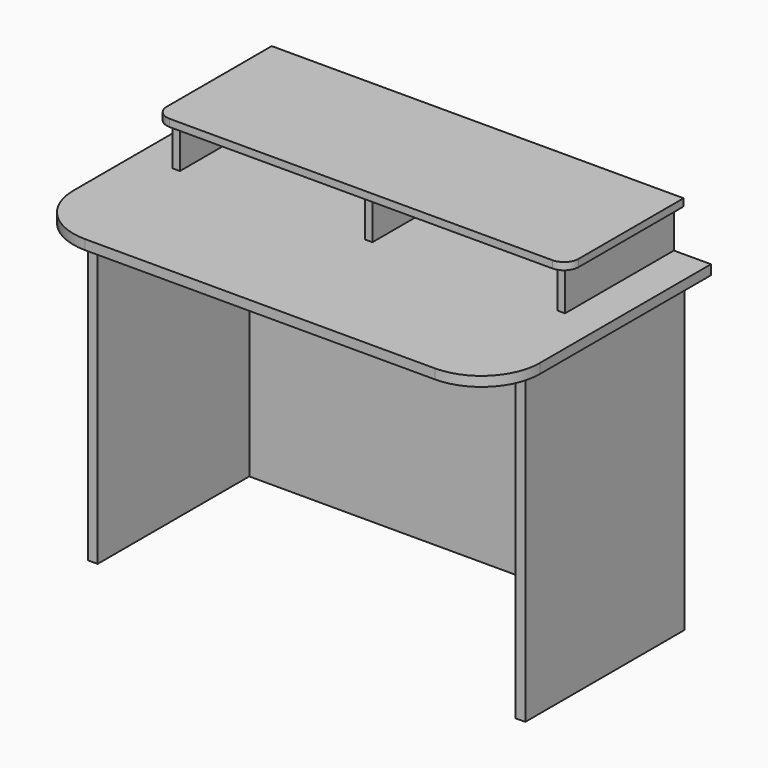
from build123d import *

# Parameters (mm, degrees)
F0_W      = 1219.2
F0_H      = 711.2
F1_DEPTH  = 25.4
F3_DEPTH  = 25.4
F4_W      = 19.05
F4_H      = 355.6
F5_DEPTH  = 109.5375
F6_W      = 1092.2
F6_H      = 25.4
F7_DEPTH  = 812.8
F8_W      = 19.05
F8_H      = 355.6
F9_DEPTH  = 19.05
F10_R     = 38.1
F11_W     = 203.2
F11_H     = 254
F12_DEPTH = 25.4
F13_R     = 25.4


# Not quite as in the source:
# - a feature names something its author has since deleted; it is built from what else it names


with BuildPart() as f1:
    # F0 (on Top) → F1 (new body)
    with BuildSketch(Plane.XY):
        with Locations((609.6, 355.6)):
            Rectangle(F0_W, F0_H)
    extrude(amount=F1_DEPTH)

    # F2 (on face) → F3 (cut)
    with BuildSketch(Plane.XY.offset(25.4)):
        with BuildLine():
            ThreePointArc((152.4, 0), (44.6369265472, 44.6369265472), (0, 152.4))
            Line((0, 152.4), (0, 0))
            Line((0, 0), (152.4, 0))
        make_face()
        with BuildLine():
            ThreePointArc((1219.2, 152.4), (1174.5630734528, 44.6369265472), (1066.8, 0))
            Line((1066.8, 0), (1219.2, 0))
            Line((1219.2, 0), (1219.2, 152.4))
        make_face()
    extrude(amount=-F3_DEPTH, mode=Mode.SUBTRACT)


with BuildPart() as f5:
    # F4 (on face) → F5 (new body)
    with BuildSketch(Plane.XY.offset(25.4)):
        with Locations((106.3625, 533.4)):
            Rectangle(F4_W, F4_H)
    extrude(amount=F5_DEPTH)


with BuildPart() as f5b:
    # F4 (on face) → F5, piece 2 (new body)
    with BuildSketch(Plane.XY.offset(25.4)):
        with Locations((609.6, 533.4)):
            Rectangle(F4_W, F4_H)
    extrude(amount=F5_DEPTH)


with BuildPart() as f5c:
    # F4 (on face) → F5, piece 3 (new body)
    with BuildSketch(Plane.XY.offset(25.4)):
        with Locations((1112.8375, 533.4)):
            Rectangle(F4_W, F4_H)
    extrude(amount=F5_DEPTH)


with BuildPart() as f7:
    # F6 (on face) → F7 (new body)
    with BuildSketch(Plane(origin=(0, 0, 0), x_dir=(1, 0, 0), z_dir=(0, 0, -1))):
        Polygon((63.5, -152.4), (38.1, -152.4), (38.1, -673.1), (63.5, -673.1), (63.5, -647.7), align=None)
        with Locations((609.6, -660.4)):
            Rectangle(F6_W, F6_H)
        Polygon((1155.7, -152.4), (1155.7, -647.7), (1155.7, -673.1), (1181.1, -673.1), (1181.1, -152.4), align=None)
    extrude(amount=F7_DEPTH)

    # F11 (on face) → F12 (cut)
    with BuildSketch(Plane.XZ.offset(-647.7)):
        with Locations((977.9, -685.8)):
            Rectangle(F11_W, F11_H)
    extrude(amount=-F12_DEPTH, mode=Mode.SUBTRACT)

    # F13
    f13_edges = [f7.edges().sort_by_distance(p)[0] for p in [
        (1079.5, 660.4, -558.8),
        (876.3, 660.4, -558.8),
    ]]
    fillet(f13_edges, radius=F13_R)


with BuildPart() as f9:
    # F8 (on face) → F9 (new body)
    with BuildSketch(Plane.XY.offset(134.9375)):
        Polygon((96.8375, 711.2), (71.4375, 711.2), (71.4375, 330.2), (1147.7625, 330.2), (1147.7625, 711.2), (115.8875, 711.2), (115.8875, 355.6), (96.8375, 355.6), align=None)
        with Locations((106.3625, 533.4)):
            Rectangle(F8_W, F8_H)
    extrude(amount=F9_DEPTH)

    # F10
    f10_edges = [f9.edges().sort_by_distance(p)[0] for p in [
        (71.4375, 330.2, 144.4625),
        (1147.7625, 330.2, 144.4625),
    ]]
    fillet(f10_edges, radius=F10_R)


solid = Compound([f1.part, f5.part, f5b.part, f5c.part, f7.part, f9.part])
